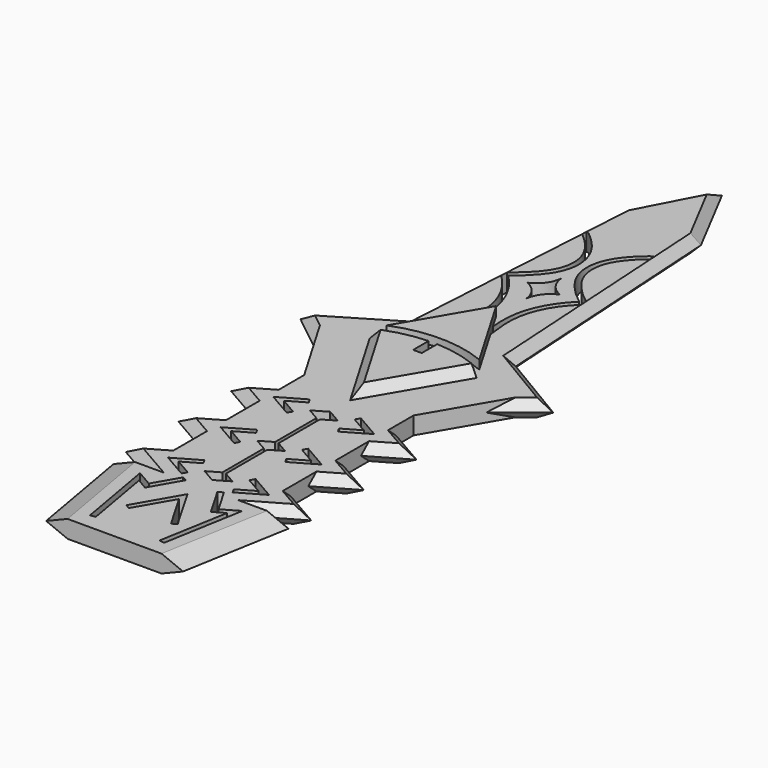
from build123d import *

# Parameters (mm, degrees)
F1_DEPTH      = 0.5
F1_DEPTH_BACK = 0.5
F2_SIZE       = 0.49999
F3_SIZE       = 0.49999
F4_T4_DEPTH   = 14.0284913346
F4_T9_DEPTH   = 14.0284913346
F4_T14_DEPTH  = 14.0284913346
F4_T19_DEPTH  = 14.0284913346
F6_DEPTH      = 1
F8_DEPTH      = 1
F8_DEPTH_BACK = 1
F9_SIZE       = 0.49999
F11_DEPTH     = 1


# Not quite as in the source:
# - a fillet or chamfer that OpenCascade refuses, or shapes differently, is made with other operations: its cross-section is extruded or revolved along the edge and cut away or added
# - a fillet or chamfer is up to 0.001 mm smaller than in the source, because OpenCascade refuses the exact size
# - ends of sketch curves that miss each other by under 0.0002 mm in the source are joined
# - the dataset's text gives a spline's control points without its knots; the knots are read off the source's solid


with BuildPart() as f1:
    # F0 (on Top) → F1 (new body, two sides)
    with BuildSketch(Plane.XY) as f1_sk:
        Polygon((2.2514325101, 39.5025983453), (0, 43.810781488), (-2.2514325101, 39.5025983453), (-3.1174682453, 25.2306121398), (-7.2010022417, 22.7936655283), (-4.8688513056, 20.9399051964), (-3.1174682453, 17.9508924671), (-3.1174682453, 16.7008924671), (-5.2825317547, 15.4508924671), (-3.1174682453, 14.2008924671), (-3.1174682453, 12.9508924671), (-5.2825317547, 11.7008924671), (-3.1174682453, 10.4508924671), (-3.1174682453, 9.2008924671), (-5.2825317547, 7.9508924671), (-3.1174682453, 6.7008924671), (-5.2825317547, 6.7008924671), (-4.2, 0.5448688171), (0, 0.5448688171), (4.2, 0.5448688171), (5.2825317547, 6.7008924671), (3.1174682453, 6.7008924671), (5.2825317547, 7.9508924671), (3.1174682453, 9.2008924671), (3.1174682453, 10.4508924671), (5.2825317547, 11.7008924671), (3.1174682453, 12.9508924671), (3.1174682453, 14.2008924671), (5.2825317547, 15.4508924671), (3.1174682453, 16.7008924671), (3.1174682453, 17.9508924671), (4.8688513056, 20.9399051964), (7.2010022417, 22.7936655283), (3.1174682453, 25.2306121398), align=None)
    extrude(amount=F1_DEPTH)
    extrude(f1_sk.sketch, amount=-F1_DEPTH_BACK)

    # F2 (size 0.5 in the source; OpenCascade refuses exactly that, so slightly less here)
    f2_edges = [f1.edges().sort_by_distance(p)[0] for p in [
        (2.68445, 32.366605, 0.5),
        (2.68445, 32.366605, -0.5),
        (1.125716, 41.65669, 0.5),
        (1.125716, 41.65669, -0.5),
        (-1.125716, 41.65669, 0.5),
        (-1.125716, 41.65669, -0.5),
        (-2.68445, 32.366605, 0.5),
        (-2.68445, 32.366605, -0.5),
        (5.159235, 24.012139, -0.5),
        (5.159235, 24.012139, 0.5),
        (6.034927, 21.866785, -0.5),
        (6.034927, 21.866785, 0.5),
        (-5.159235, 24.012139, 0.5),
        (-5.159235, 24.012139, -0.5),
        (-6.034927, 21.866785, 0.5),
        (-6.034927, 21.866785, -0.5),
    ]]
    chamfer(f2_edges, length=F2_SIZE)

    # F3 (size 0.5 in the source; OpenCascade refuses exactly that, so slightly less here)
    f3_edges = [f1.edges().sort_by_distance(p)[0] for p in [
        (-4.2, 16.075892, 0.5),
        (-4.2, 14.825892, 0.5),
        (-4.2, 12.325892, 0.5),
        (-4.2, 11.075892, 0.5),
        (-4.2, 8.575892, 0.5),
        (-4.2, 7.325892, 0.5),
        (-4.2, 16.075892, -0.5),
        (-4.2, 14.825892, -0.5),
        (-4.2, 12.325892, -0.5),
        (-4.2, 11.075892, -0.5),
        (-4.2, 8.575892, -0.5),
        (-4.2, 7.325892, -0.5),
        (4.2, 16.075892, -0.5),
        (4.2, 16.075892, 0.5),
        (4.2, 14.825892, 0.5),
        (4.2, 14.825892, -0.5),
        (4.2, 12.325892, -0.5),
        (4.2, 12.325892, 0.5),
        (4.2, 11.075892, 0.5),
        (4.2, 11.075892, -0.5),
        (4.2, 8.575892, 0.5),
        (4.2, 8.575892, -0.5),
        (4.2, 7.325892, 0.5),
        (4.2, 7.325892, -0.5),
    ]]
    chamfer(f3_edges, length=F3_SIZE)

    # F4: chamfer of 1.5 x 0.6213203436 on 4 edges, made by hand


with BuildPart() as f4_tool2:
    # F4_s3 → F4_t4 (new body)
    with BuildSketch(Plane(origin=(-1.9749969173, 11.2311973098, 0), x_dir=(0, 0, 1), z_dir=(0.1731917753, -0.98488812, 0))):
        Polygon((0.5, 2.5421633064), (-0.1213203436, 4.0421633064), (0.5, 4.0421633064), align=None)
    extrude(amount=F4_T4_DEPTH)

    split(bisect_by=Plane(origin=(2.1222044909, 3.6757660023, 0), x_dir=(0, 0, 1), z_dir=(-0.5, -0.8660254038, 0)), keep=Keep.TOP)


with BuildPart() as f1_1:
    add(f1.part)

    # F4_t1: cut F4_tool2
    add(f4_tool2.part, mode=Mode.SUBTRACT)


with BuildPart() as f4_tool7:
    # F4_s8 → F4_t9 (new body)
    with BuildSketch(Plane(origin=(-1.9749969173, 11.2311973098, 0), x_dir=(0, 0, 1), z_dir=(0.1731917753, -0.98488812, 0))):
        Polygon((0.1213203436, 4.0421633064), (-0.5, 2.5421633064), (-0.5, 4.0421633064), align=None)
    extrude(amount=F4_T9_DEPTH)

    split(bisect_by=Plane(origin=(1.0610997455, 1.837878671, 2.1221994909), x_dir=(0.8660254038, -0.5, 0), z_dir=(-0.3535533906, -0.6123724357, -0.7071067812)), keep=Keep.TOP)


with BuildPart() as f1_2:
    add(f1_1.part)

    # F4_t6: cut F4_tool7
    add(f4_tool7.part, mode=Mode.SUBTRACT)


with BuildPart() as f4_tool12:
    # F4_s13 → F4_t14 (new body)
    with BuildSketch(Plane(origin=(-0.4546224018, -2.5852971475, 0), x_dir=(0, 0, 1), z_dir=(0.1731917753, 0.98488812, 0))):
        Polygon((0.1213203436, 4.0421633064), (-0.5, 2.5421633064), (-0.5, 4.0421633064), align=None)
    extrude(amount=F4_T14_DEPTH)

    split(bisect_by=Plane(origin=(-1.0610997455, 1.837878671, 2.1221994909), x_dir=(0.8660254038, 0.5, 0), z_dir=(0.3535533906, -0.6123724357, -0.7071067812)), keep=Keep.TOP)


with BuildPart() as f1_3:
    add(f1_2.part)

    # F4_t11: cut F4_tool12
    add(f4_tool12.part, mode=Mode.SUBTRACT)


with BuildPart() as f4_tool17:
    # F4_s18 → F4_t19 (new body)
    with BuildSketch(Plane(origin=(-0.4546224018, -2.5852971475, 0), x_dir=(0, 0, 1), z_dir=(0.1731917753, 0.98488812, 0))):
        Polygon((0.5, 2.5421633064), (-0.1213203436, 4.0421633064), (0.5, 4.0421633064), align=None)
    extrude(amount=F4_T19_DEPTH)

    split(bisect_by=Plane(origin=(-2.1222044909, 3.6757660023, 0), x_dir=(0, 0, 1), z_dir=(0.5, -0.8660254038, 0)), keep=Keep.TOP)


with BuildPart() as f1_4:
    add(f1_3.part)

    # F4_t16: cut F4_tool17
    add(f4_tool17.part, mode=Mode.SUBTRACT)

    # F5 (on face) → F6 (cut)
    with BuildSketch(Plane.XY.offset(0.5)):
        Polygon((-2.9182584163, 6.0045817738), (-2.113919944, 1.4305573754), (-1.818453508, 1.482514908), (-2.5114360649, 5.4232926182), (-1.874469753, 5.0555399465), (-0.9023789929, 6.7392505326), (-1.162186614, 6.8892505326), (-1.9842773741, 5.4653475677), align=None)
        Polygon((0, 5.742299924), (-1.4604201439, 3.2127780344), (-1.2006125228, 3.0627780344), (0, 5.142299924), (1.2006125228, 3.0627780344), (1.4604201439, 3.2127780344), align=None)
        Polygon((-2.8771683473, 7.9508924671), (-1.4582556271, 7.1316828261), (-1.3082556271, 7.3914904472), (-2.2771683473, 7.9508924671), (-1.3082556271, 8.5102944869), (-1.4582556271, 8.770102108), align=None)
        Polygon((-2.8771683473, 11.7008924671), (-1.4582556271, 10.8816828261), (-1.3082556271, 11.1414904472), (-2.2771683473, 11.7008924671), (-1.3082556271, 12.2602944869), (-1.4582556271, 12.520102108), align=None)
        Polygon((-2.8771683473, 15.4508924671), (-1.4582556271, 14.6316828261), (-1.3082556271, 14.8914904472), (-2.2771683473, 15.4508924671), (-1.3082556271, 16.0102944869), (-1.4582556271, 16.270102108), align=None)
        Polygon((2.2771683473, 15.4508924671), (1.3082556271, 14.8914904472), (1.4582556271, 14.6316828261), (2.8771683473, 15.4508924671), (1.4582556271, 16.270102108), (1.3082556271, 16.0102944869), align=None)
        Polygon((2.2771683473, 7.9508924671), (1.3082556271, 7.3914904472), (1.4582556271, 7.1316828261), (2.8771683473, 7.9508924671), (1.4582556271, 8.770102108), (1.3082556271, 8.5102944869), align=None)
        Polygon((2.8771683473, 11.7008924671), (1.4582556271, 12.520102108), (1.3082556271, 12.2602944869), (2.2771683473, 11.7008924671), (1.3082556271, 11.1414904472), (1.4582556271, 10.8816828261), align=None)
        Polygon((1.818453508, 1.482514908), (2.113919944, 1.4305573754), (2.9182584163, 6.0045817738), (1.9842773741, 5.4653475677), (1.162186614, 6.8892505326), (0.9023789929, 6.7392505326), (1.874469753, 5.0555399465), (2.5114360649, 5.4232926182), align=None)
        Polygon((-0.7935423827, 7.9508924671), (0, 7.4927405588), (0.7935423827, 7.9508924671), (0.1, 8.3513093484), (0, 8.4090443753), (-0.1, 8.3513093484), align=None)
        Polygon((-0.1, 11.3004755857), (-0.1, 8.3513093484), (0, 8.4090443753), (0.1, 8.3513093484), (0.1, 11.3004755857), (0, 11.2427405588), align=None)
        Polygon((-0.7935423827, 11.7008924671), (-0.1, 11.3004755857), (0, 11.2427405588), (0.1, 11.3004755857), (0.7935423827, 11.7008924671), (0.1, 12.1013093484), (0, 12.1590443753), (-0.1, 12.1013093484), align=None)
        Polygon((-0.1, 15.0504755857), (-0.1, 12.1013093484), (0, 12.1590443753), (0.1, 12.1013093484), (0.1, 15.0504755857), (0, 14.9927405588), align=None)
        Polygon((-0.7935423827, 15.4508924671), (-0.1, 15.0504755857), (0, 14.9927405588), (0.1, 15.0504755857), (0.7935423827, 15.4508924671), (0, 15.9090443753), align=None)
    extrude(amount=-F6_DEPTH, mode=Mode.SUBTRACT)

    # F7 (on Top) → F8 (join, two sides)
    with BuildSketch(Plane.XY) as f8_sk:
        with BuildLine():
            ThreePointArc((-2.639605651, 23.2251665721), (0, 23.7415439887), (2.639605651, 23.2251665721))
            Line((2.639605651, 23.2251665721), (0, 27.7300719066))
            Line((0, 27.7300719066), (-2.639605651, 23.2251665721))
        make_face()
        with BuildLine():
            Line((-3.0487553833, 22.526887717), (0, 17.3237035273))
            Line((0, 17.3237035273), (3.0487553833, 22.526887717))
            ThreePointArc((3.0487553833, 22.526887717), (1.682776579, 23.0200323923), (0.244464298, 23.2208993809))
            Line((0.244464298, 23.2208993809), (0.244464298, 22.1209414064))
            Line((0.244464298, 22.1209414064), (0, 22.1209414064))
            Line((0, 22.1209414064), (-0.244464298, 22.1209414064))
            Line((-0.244464298, 22.1209414064), (-0.244464298, 23.2208993809))
            ThreePointArc((-0.244464298, 23.2208993809), (-1.682776579, 23.0200323923), (-3.0487553833, 22.526887717))
        make_face()
    extrude(amount=F8_DEPTH)
    extrude(f8_sk.sketch, amount=-F8_DEPTH_BACK)

    # F9 (size 0.5 in the source; OpenCascade refuses exactly that, so slightly less here)
    f9_edges = [f1_4.edges().sort_by_distance(p)[0] for p in [
        (1.524378, 19.925296, 1),
        (-1.524378, 19.925296, 1),
        (-1.524378, 19.925296, -1),
        (1.524378, 19.925296, -1),
    ]]
    chamfer(f9_edges, length=F9_SIZE)

    # F10 (on face) → F11 (cut)
    with BuildSketch(Plane.XY.offset(0.5)):
        with BuildLine():
            add(Edge.make_bspline(
                [(0.5240877447, 26.8354920593), (0.5024381397, 27.0566155827), (0.4734613578, 27.4860732933), (0.4934729621, 28.1130059743), (0.6362710333, 28.9500865377), (1.0657658408, 29.9982471602), (1.6697042342, 30.7663254033), (2.0304100579, 31.1086318926)],
                knots=[0.1252998939, 0.1252998939, 0.1252998939, 0.1252998939, 0.25, 0.375, 0.5, 0.75, 0.991945534, 0.991945534, 0.991945534, 0.991945534], degree=3))
            Line((0.5240877447, 26.8354920593), (0.904888709, 26.1857359295))
            add(Edge.make_bspline(
                [(0.904888709, 26.1857359295), (0.7785311686, 27.1073159917), (0.6472574871, 28.6199331355), (1.5399421957, 30.242128838), (2.2711191384, 30.923176094)],
                knots=[0, 0, 0, 0, 0.4864024509, 1, 1, 1, 1], degree=3))
            Line((2.2711191384, 30.923176094), (2.246938872, 31.3216589912))
            add(Edge.make_bspline(
                [(2.246938872, 31.3216589912), (1.7577497369, 31.680175135), (0.8504112125, 32.5489054376), (0.323244609, 34.0155843801), (0.8153166273, 35.3659763932), (1.9459843851, 36.2812906903)],
                knots=[0, 0, 0, 0, 0.3239944256, 0.6017145977, 1, 1, 1, 1], degree=3))
            Line((1.9459843851, 36.2812906903), (1.9278135642, 36.5807398868))
            Line((1.9278135642, 36.5807398868), (1.7572234432, 36.5144629588))
            add(Edge.make_bspline(
                [(2.0304100579, 31.1086318926), (1.8458079926, 31.2460268158), (1.4661770597, 31.559509272), (0.9443536757, 32.1000661237), (0.5252644806, 32.6908097171), (0.310267521, 33.2188895151), (0.2332324505, 33.6737974602), (0.2202737855, 34.1461209238), (0.3410138753, 34.7982987514), (0.8106725709, 35.6336128143), (1.3877476498, 36.2153596425), (1.7572234432, 36.5144629588)],
                knots=[0.0082581177, 0.0082581177, 0.0082581177, 0.0082581177, 0.125, 0.25, 0.375, 0.5, 0.5625, 0.625, 0.75, 0.875, 1, 1, 1, 1], degree=3))
        make_face()
        with BuildLine():
            add(Edge.make_bspline(
                [(-0.904888709, 26.1857359295), (-0.7785311686, 27.1073159917), (-0.6472574871, 28.6199331355), (-1.5399421957, 30.242128838), (-2.2711191384, 30.923176094)],
                knots=[0, 0, 0, 0, 0.4864024509, 1, 1, 1, 1], degree=3))
            Line((-0.904888709, 26.1857359295), (-0.5241659133, 26.8354997125))
            add(Edge.make_bspline(
                [(-0.5241659133, 26.8354997125), (-0.5024381397, 27.0566155827), (-0.4734613578, 27.4860732933), (-0.4934729621, 28.1130059743), (-0.6362710333, 28.9500865377), (-1.0657658408, 29.9982471602), (-1.6697042342, 30.7663254033), (-2.0304100579, 31.1086318926)],
                knots=[0.1252998939, 0.1252998939, 0.1252998939, 0.1252998939, 0.25, 0.375, 0.5, 0.75, 0.991945534, 0.991945534, 0.991945534, 0.991945534], degree=3))
            add(Edge.make_bspline(
                [(-2.0304100579, 31.1086318926), (-1.8458079926, 31.2460268158), (-1.4661770597, 31.559509272), (-0.9443536757, 32.1000661237), (-0.5252644806, 32.6908097171), (-0.310267521, 33.2188895151), (-0.2332324505, 33.6737974602), (-0.2202737855, 34.1461209238), (-0.3410138753, 34.7982987514), (-0.8106725709, 35.6336128143), (-1.3877476498, 36.2153596425), (-1.7572234432, 36.5144629588)],
                knots=[0.0082581177, 0.0082581177, 0.0082581177, 0.0082581177, 0.125, 0.25, 0.375, 0.5, 0.5625, 0.625, 0.75, 0.875, 1, 1, 1, 1], degree=3))
            Line((-1.7572234432, 36.5144629588), (-1.9278135642, 36.5807398868))
            Line((-1.9278135642, 36.5807398868), (-1.9459843851, 36.2812906903))
            add(Edge.make_bspline(
                [(-2.246938872, 31.3216589912), (-1.7577497369, 31.680175135), (-0.8504112125, 32.5489054376), (-0.323244609, 34.0155843801), (-0.8153166273, 35.3659763932), (-1.9459843851, 36.2812906903)],
                knots=[0, 0, 0, 0, 0.3239944256, 0.6017145977, 1, 1, 1, 1], degree=3))
            Line((-2.246938872, 31.3216589912), (-2.2711191384, 30.923176094))
        make_face()
        with BuildLine():
            ThreePointArc((0, 32.3459384355), (-0.2933356502, 31.5987059912), (-0.9291260097, 31.108631764))
            ThreePointArc((-0.9291260097, 31.108631764), (-0.2933356502, 30.6185575367), (0, 29.8713250925))
            ThreePointArc((0, 29.8713250925), (0.2933356502, 30.6185575367), (0.9291260097, 31.108631764))
            ThreePointArc((0.9291260097, 31.108631764), (0.2933356502, 31.5987059912), (0, 32.3459384355))
        make_face()
    extrude(amount=-F11_DEPTH, mode=Mode.SUBTRACT)


solid = f1_4.part
